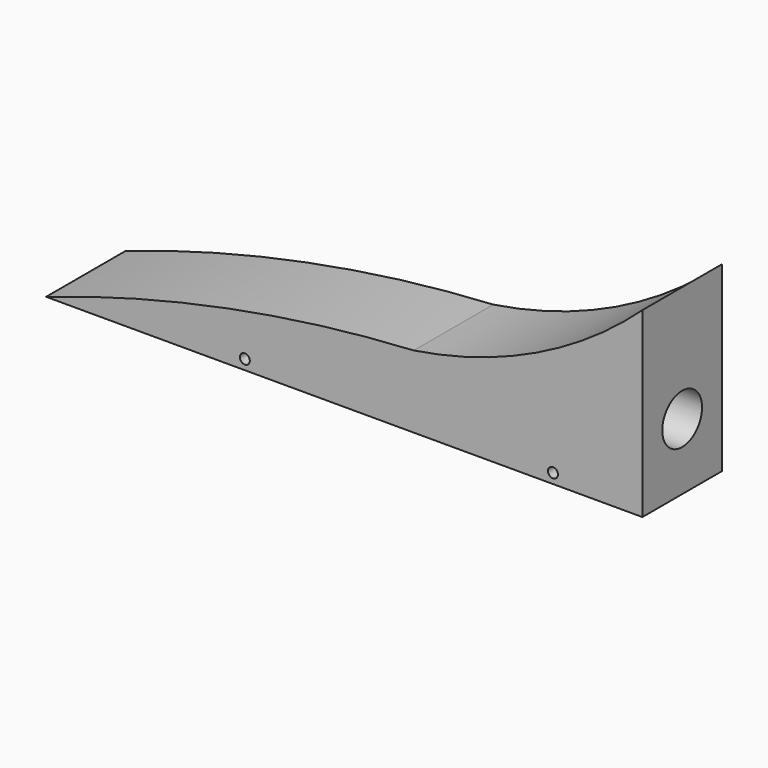
from build123d import *

# Parameters (mm, degrees)
F1_DEPTH = 38.1
F2_R     = 5.08
F3_DEPTH = 38.1
F4_R     = 9.525
F5_DEPTH = 53.34
F6_R     = 1.905
F7_DEPTH = 38.101
F8_DEPTH = 38.101


# Not quite as in the source:
# - a feature names something its author has since deleted; it is built from what else it names


with BuildPart() as f1:
    # F0 (on Front) → F1 (new body)
    with BuildSketch(Plane.XZ):
        with BuildLine():
            ThreePointArc((140.9522952768, 27.729119938), (69.5233725404, 18.7076937305), (0, 0))
            Line((0, 0), (228.6, 0))
            Line((228.6, 0), (228.6, 25.4))
            ThreePointArc((228.6, 25.4), (184.8248483375, 28.3972283618), (140.9522952768, 27.729119938))
        make_face()
    extrude(amount=F1_DEPTH)

    # F2
    f2_edges = [f1.edges().sort_by_distance(p)[0] for p in [
        (112.892107, 0, 25.371039),
        (112.892107, -38.1, 25.371039),
    ]]
    fillet(f2_edges, radius=F2_R)

    # F0 (on Front) → F3 (join)
    with BuildSketch(Plane.XZ):
        with BuildLine():
            ThreePointArc((140.9522952768, 27.729119938), (69.5233725404, 18.7076937305), (0, 0))
            Line((0, 0), (228.6, 0))
            Line((228.6, 0), (228.6, 25.4))
            ThreePointArc((228.6, 25.4), (184.8248483375, 28.3972283618), (140.9522952768, 27.729119938))
        make_face()
        with BuildLine():
            ThreePointArc((228.6, 69.85), (187.9185150392, 42.2507295914), (140.9522952768, 27.729119938))
            ThreePointArc((140.9522952768, 27.729119938), (184.8248483375, 28.3972283618), (228.6, 25.4))
            Line((228.6, 25.4), (228.6, 69.85))
        make_face()
    extrude(amount=F3_DEPTH)

    # F4 (on face) → F5 (cut)
    with BuildSketch(Plane.YZ.offset(228.6)):
        with Locations((-19.05, 25.4)):
            Circle(F4_R)
    extrude(amount=-F5_DEPTH, mode=Mode.SUBTRACT)

    # F6 (on face) → F7 (cut, through all)
    with BuildSketch(Plane.XZ.offset(38.1)):
        with Locations((76.2, 3.81)):
            Circle(F6_R)
    extrude(amount=-F7_DEPTH, mode=Mode.SUBTRACT)

    # F6 (on face) → F8 (cut, through all)
    with BuildSketch(Plane.XZ.offset(38.1)):
        with Locations((194.31, 3.81)):
            Circle(F6_R)
    extrude(amount=-F8_DEPTH, mode=Mode.SUBTRACT)


solid = f1.part
